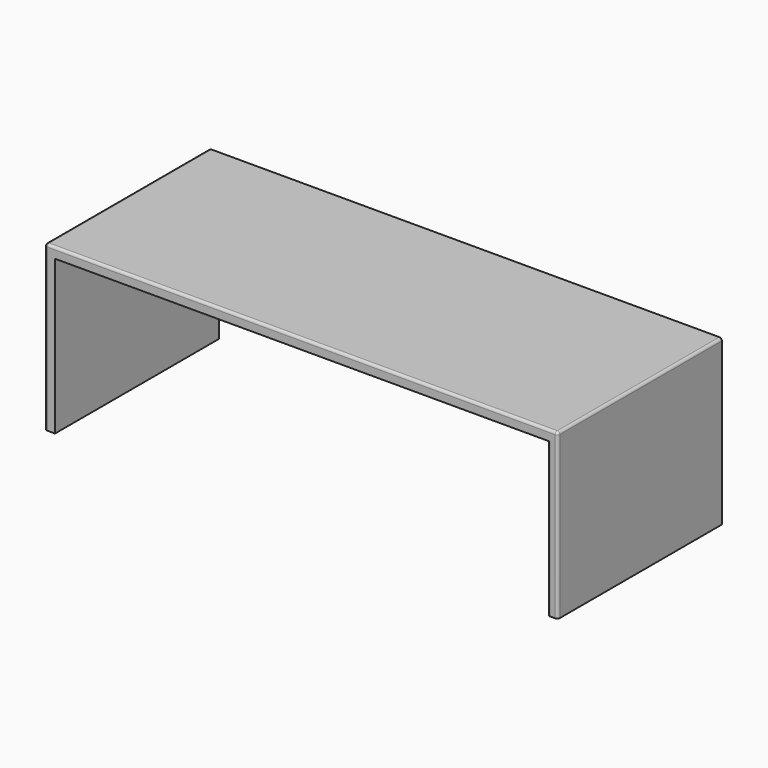
from build123d import *

# Parameters (mm, degrees)
F0_W     = 1000
F0_H     = 400
F1_DEPTH = 20
F2_W     = 20
F2_H     = 400
F3_DEPTH = 300
F4_R     = 5
F5_R     = 5
F6_R     = 5


with BuildPart() as f1:
    # F0 (on Top) → F1 (new body)
    with BuildSketch(Plane.XY):
        with Locations((-78.8800735027, -73.4630868891)):
            Rectangle(F0_W, F0_H)
    extrude(amount=F1_DEPTH)

    # F2 (on face) → F3 (join)
    with BuildSketch(Plane.XY):
        with Locations((-568.8800735027, -73.4630868891)):
            Rectangle(F2_W, F2_H)
        with Locations((411.1199264973, -73.4630868891)):
            Rectangle(F2_W, F2_H)
    extrude(amount=-F3_DEPTH)

    # F4
    f4_edges = [f1.edges().sort_by_distance(p)[0] for p in [
        (-78.880074, -273.463087, 20),
    ]]
    fillet(f4_edges, radius=F4_R)

    # F5
    f5_edges = [f1.edges().sort_by_distance(p)[0] for p in [
        (421.119926, -70.963087, 20),
    ]]
    fillet(f5_edges, radius=F5_R)

    # F6
    f6_edges = [f1.edges().sort_by_distance(p)[0] for p in [
        (401.119926, -273.463087, -150),
        (-578.880074, -70.963087, 20),
    ]]
    fillet(f6_edges, radius=F6_R)


solid = f1.part
